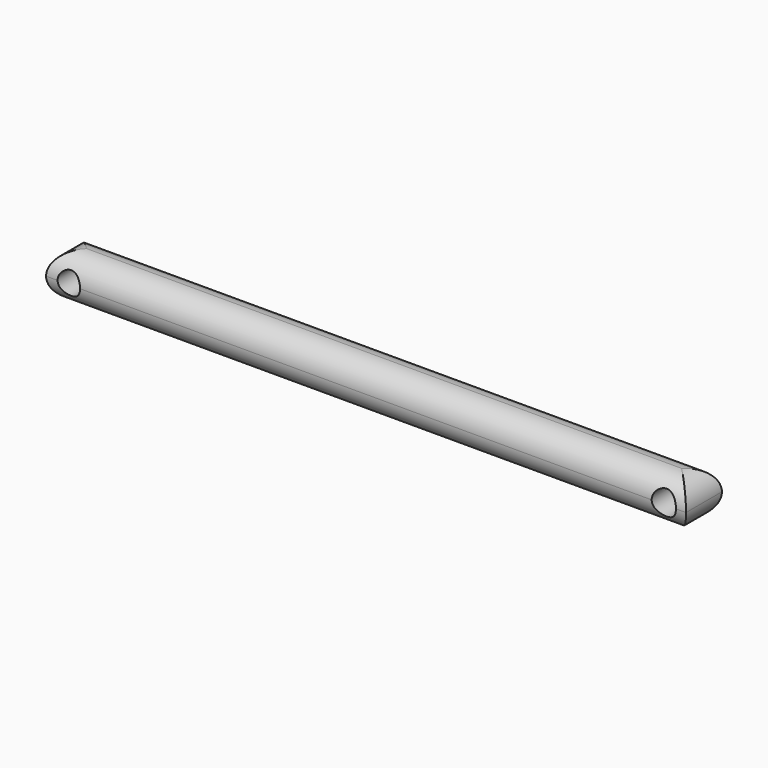
from build123d import *

# Parameters (mm, degrees)
F0_W     = 285
F0_H     = 20
F1_DEPTH = 20
F2_R     = 9.99999
F3_R     = 5
F3_R_2   = 5.4133078472
F4_DEPTH = 20


# Not quite as in the source:
# - a fillet or chamfer is up to 0.001 mm smaller than in the source, because OpenCascade refuses the exact size


with BuildPart() as f1:
    # F0 (on Front) → F1 (new body)
    with BuildSketch(Plane.XZ):
        with Locations((-142.5, 10)):
            Rectangle(F0_W, F0_H)
    extrude(amount=F1_DEPTH)

    # F2 (radius 10 in the source; OpenCascade refuses exactly that, so slightly less here)
    f2_edges = [f1.edges().sort_by_distance(p)[0] for p in [
        (-142.5, -20, 20),
        (-142.5, 0, 20),
        (-142.5, -20, 0),
        (0, -10, 0),
        (-142.5, 0, 0),
        (-285, -10, 0),
        (0, -10, 20),
        (-285, -10, 20),
    ]]
    fillet(f2_edges, radius=F2_R)

    # F3 (on Front) → F4 (cut)
    with BuildSketch(Plane.XZ):
        with Locations((-274.8824357986, 10.0639369339)):
            Circle(F3_R)
        with Locations((-9.8824357986, 10.070726499)):
            Circle(F3_R_2)
    extrude(amount=F4_DEPTH, mode=Mode.SUBTRACT)


solid = f1.part
